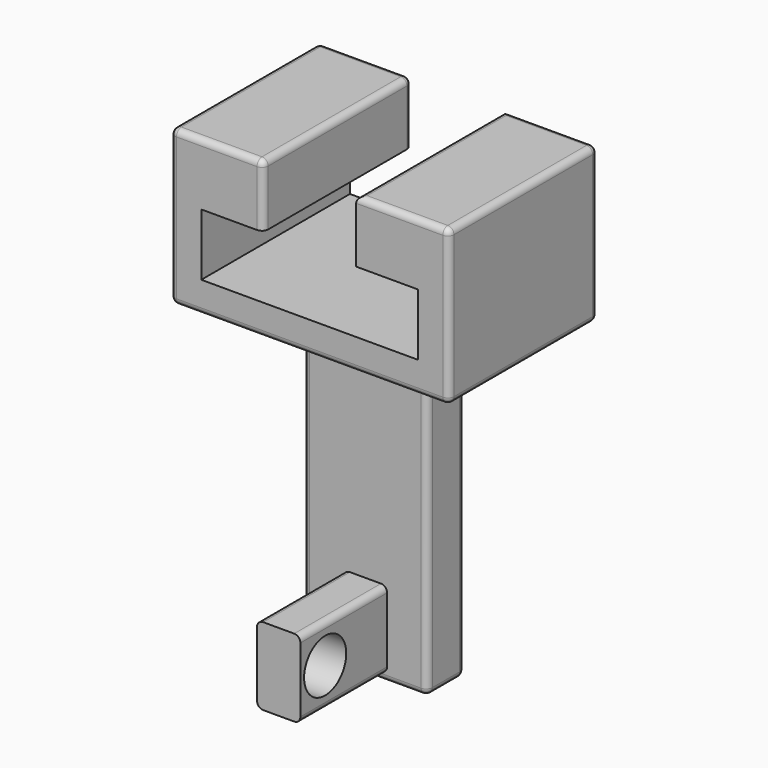
from build123d import *

# Parameters (mm, degrees)
F0_W      = 90
F0_H      = 60
F1_DEPTH  = 10
F2_W      = 10
F2_H      = 60
F3_DEPTH  = 20
F5_W      = 30
F5_H      = 60
F6_DEPTH  = 20
F4_W      = 30
F4_H      = 60
F7_DEPTH  = 20
F8_W      = 40
F8_H      = 15
F9_DEPTH  = 100
F10_W     = 14
F10_H     = 25
F11_DEPTH = 50
F12_R     = 8.5
F13_DEPTH = 52.001
F14_R     = 2


with BuildPart() as f1:
    # F0 (on Top) → F1 (new body)
    with BuildSketch(Plane.XY):
        Rectangle(F0_W, F0_H)
    extrude(amount=F1_DEPTH)

    # F2 (on face) → F3 (join)
    with BuildSketch(Plane.XY.offset(10)):
        with Locations((-40, 0)):
            Rectangle(F2_W, F2_H)
        with Locations((40, 0)):
            Rectangle(F2_W, F2_H)
    extrude(amount=F3_DEPTH)

    # F5 (on face) → F6 (join)
    with BuildSketch(Plane.XY.offset(30)):
        with Locations((30, 0)):
            Rectangle(F5_W, F5_H)
    extrude(amount=F6_DEPTH)

    # F4 (on face) → F7 (join)
    with BuildSketch(Plane.XY.offset(30)):
        with Locations((-30, 0)):
            Rectangle(F4_W, F4_H)
    extrude(amount=F7_DEPTH)

    # F8 (on face) → F9 (join)
    with BuildSketch(Plane(origin=(0, 0, 0), x_dir=(1, 0, 0), z_dir=(0, 0, -1))):
        Rectangle(F8_W, F8_H)
    extrude(amount=F9_DEPTH)

    # F10 (on face) → F11 (join)
    with BuildSketch(Plane(origin=(0, 7.5, 0), x_dir=(-1, 0, 0), z_dir=(0, 1, 0))):
        with Locations((0, -85)):
            Rectangle(F10_W, F10_H)
    extrude(amount=-F11_DEPTH)

    # F12 (on face) → F13 (cut, through all)
    with BuildSketch(Plane(origin=(-7, 0, 0), x_dir=(0, -1, 0), z_dir=(-1, 0, 0))):
        with Locations((32.5, -85)):
            Circle(F12_R)
    extrude(amount=-F13_DEPTH, mode=Mode.SUBTRACT)

    # F14
    f14_edges = [f1.edges().sort_by_distance(p)[0] for p in [
        (-20, 7.5, -50),
        (0, 7.5, -100),
        (20, 7.5, -50),
        (20, 0, -100),
        (-20, 0, -100),
        (-20, -7.5, -50),
        (20, -7.5, -50),
        (20, 0, 0),
        (0, -7.5, -100),
        (0, 30, 0),
        (45, 30, 25),
        (30, 30, 50),
        (-15, 30, 40),
        (-30, 30, 50),
        (-45, 30, 25),
        (-45, 0, 0),
        (-45, 0, 50),
        (-45, -30, 25),
        (0, -30, 0),
        (45, 0, 0),
        (45, -30, 25),
        (45, 0, 50),
        (30, -30, 50),
        (-15, -30, 40),
        (-30, -30, 50),
        (-15, 0, 50),
        (15, 0, 50),
        (-7, -25, -97.5),
        (-7, -25, -72.5),
        (7, -25, -97.5),
        (7, -25, -72.5),
        (0, 7.5, 0),
        (-20, 0, 0),
        (0, -7.5, 0),
    ]]
    fillet(f14_edges, radius=F14_R)


solid = f1.part
